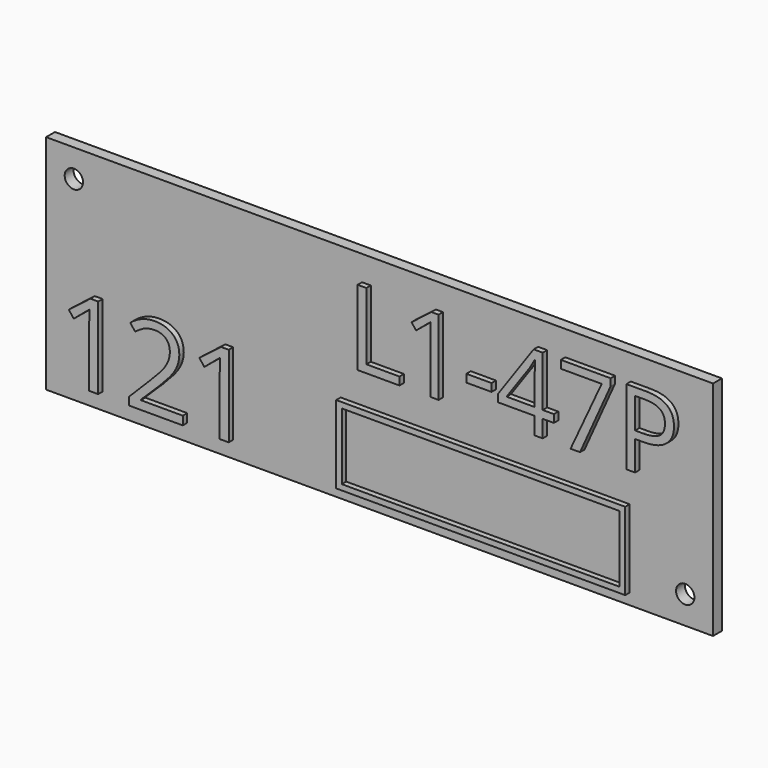
from build123d import *

# Parameters (mm, degrees)
F0_W         = 120
F0_H         = 40
F1_DEPTH     = 2
F3_D         = 3.3
F4_TEXT_SIZE = 18.9181200118
F5_DEPTH     = 1
F6_TEXT_SIZE = 20.5478077656
F7_DEPTH     = 1
F8_W         = 52
F8_H         = 14
F8_W_2       = 49.99999962
F8_H_2       = 11.99999962
F9_DEPTH     = 1


# Not quite as in the source:
# - Text() gives the source's letters only with a copy of the font that has no kerning and outlines rounded to 1/6400 em; it was checked with that copy


with BuildPart() as f1:
    # F0 (on Front) → F1 (new body)
    with BuildSketch(Plane.XZ):
        Rectangle(F0_W, F0_H)
    extrude(amount=F1_DEPTH)

    # F3 (through all)
    with Locations(Plane.XZ.offset(2)):
        with Locations((-55, 15), (55, -15)):
            Hole(F3_D / 2)

    # F4 (on face) → F5 (join)
    with BuildSketch(Plane.XZ.offset(2)):
        with Locations((-5, 2)):
            Text('L1-47P', F4_TEXT_SIZE, font='Open Sans', text_align=(TextAlign.LEFT, TextAlign.BOTTOM))
    extrude(amount=F5_DEPTH)

    # F6 (on face) → F7 (join)
    with BuildSketch(Plane.XZ.offset(2)):
        with Locations((-57, -17)):
            Text('121', F6_TEXT_SIZE, font='Open Sans', text_align=(TextAlign.LEFT, TextAlign.BOTTOM))
    extrude(amount=F7_DEPTH)

    # F8 (on face) → F9 (join)
    with BuildSketch(Plane.XZ.offset(2)):
        with Locations((19, -11)):
            Rectangle(F8_W, F8_H)
        with Locations((19, -11)):
            Rectangle(F8_W_2, F8_H_2, mode=Mode.SUBTRACT)
    extrude(amount=F9_DEPTH)


solid = f1.part
